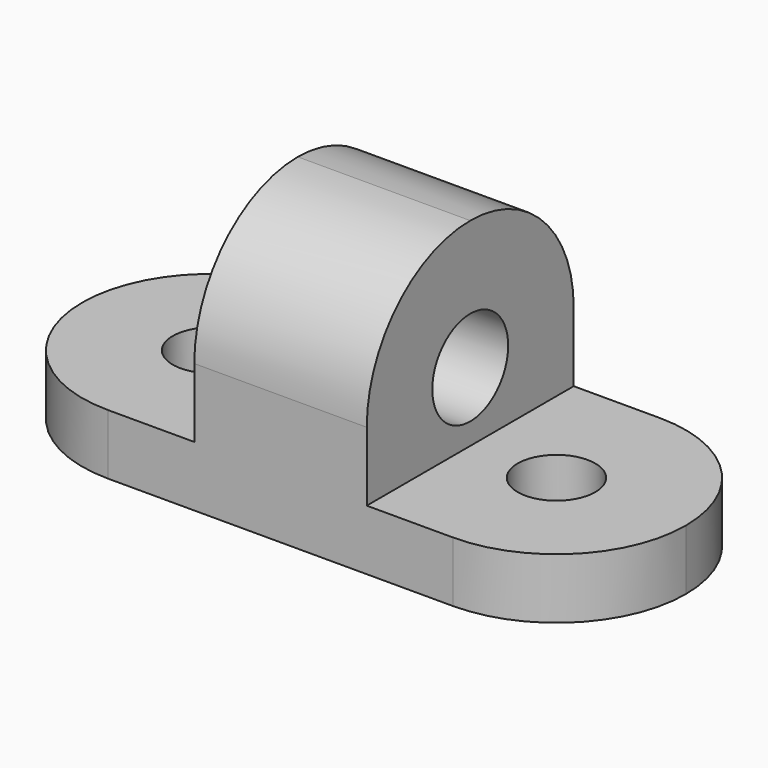
from build123d import *

# Parameters (mm, degrees)
F0_W      = 3556
F0_H      = 1524
F1_DEPTH  = 355.6
F2_W      = 1016
F2_H      = 1524
F3_DEPTH  = 1168.4
F4_R      = 761.99999
F5_R      = 279.4
F6_DEPTH  = 1016
F7_R      = 228.6
F8_DEPTH  = 355.6
F9_R      = 228.6
F10_DEPTH = 355.6


# Not quite as in the source:
# - a fillet or chamfer is up to 0.001 mm smaller than in the source, because OpenCascade refuses the exact size


with BuildPart() as f1:
    # F0 (on Top) → F1 (new body)
    with BuildSketch(Plane.XY):
        with Locations((-1778, 762)):
            Rectangle(F0_W, F0_H)
    extrude(amount=F1_DEPTH)

    # F2 (on face) → F3 (join)
    with BuildSketch(Plane.XY.offset(355.6)):
        with Locations((-1778, 762)):
            Rectangle(F2_W, F2_H)
    extrude(amount=F3_DEPTH)

    # F4 (radius 762 in the source; OpenCascade refuses exactly that, so slightly less here)
    f4_edges = [f1.edges().sort_by_distance(p)[0] for p in [
        (-1778, 0, 1524),
        (0, 0, 177.8),
        (0, 1524, 177.8),
        (-3556, 0, 177.8),
        (-3556, 1524, 177.8),
        (-1778, 1524, 1524),
    ]]
    fillet(f4_edges, radius=F4_R)

    # F5 (on face) → F6 (cut)
    with BuildSketch(Plane(origin=(-2286, 0, 0), x_dir=(0, -1, 0), z_dir=(-1, 0, 0))):
        with Locations((-762, 762)):
            Circle(F5_R)
    extrude(amount=-F6_DEPTH, mode=Mode.SUBTRACT)

    # F7 (on face) → F8 (cut)
    with BuildSketch(Plane.XY.offset(355.6)):
        with Locations((-762, 762)):
            Circle(F7_R)
    extrude(amount=-F8_DEPTH, mode=Mode.SUBTRACT)

    # F9 (on face) → F10 (cut)
    with BuildSketch(Plane.XY.offset(355.6)):
        with Locations((-2794, 762)):
            Circle(F9_R)
    extrude(amount=-F10_DEPTH, mode=Mode.SUBTRACT)


solid = f1.part
